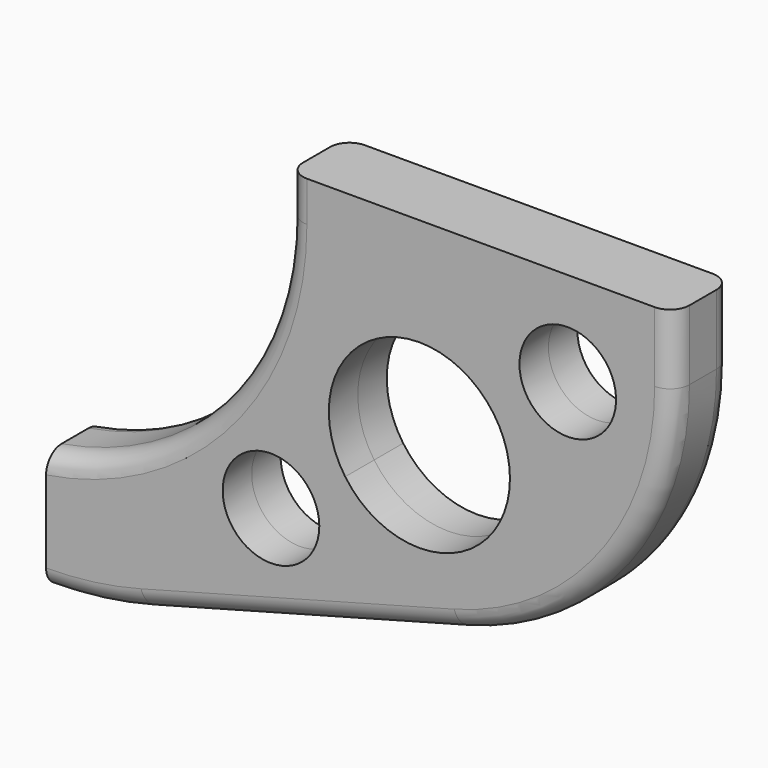
from build123d import *

# Parameters (mm, degrees)
F1_DEPTH = 9.525
F2_R     = 5.08


# Not quite as in the source:
# - a feature names something its author has since deleted; it is built from what else it names


with BuildPart() as f1:
    # F0 (on Front) → F1 (new body, symmetric)
    with BuildSketch(Plane.XZ):
        with BuildLine():
            Line((0, 15.875), (0, 0))
            ThreePointArc((0, 0), (13.2614611296, 0.8692020844), (26.2960149824, 3.461936049))
            Line((26.2960149824, 3.461936049), (108.6220112368, 25.5211202615))
            ThreePointArc((108.6220112368, 25.5211202615), (149.3535245302, 52.7370473342), (165.1, 99.1246682247))
            Line((165.1, 99.1246682247), (165.1, 117.475))
            Line((165.1, 117.475), (63.5, 117.475))
            Line((63.5, 117.475), (63.5, 106.8842132454))
            ThreePointArc((63.5, 106.8842132454), (45.4987113259, 57.6973247485), (0, 31.75))
            Line((0, 31.75), (0, 15.875))
        make_face()
        with BuildLine():
            ThreePointArc((71.8357677815, 38.1), (47.023562507, 34.2810363463), (69.5389987439, 45.3844207417))
            ThreePointArc((69.5389987439, 45.3844207417), (71.247973056, 41.9189636537), (71.8357677815, 38.1))
        make_face(mode=Mode.SUBTRACT)
        with BuildLine():
            ThreePointArc((117.6539419454, 79.0748666718), (120.8582687804, 72.5771346319), (121.9603838907, 65.4165777812))
            ThreePointArc((121.9603838907, 65.4165777812), (105.3084407414, 42.7061928915), (78.6418258361, 51.7582888906))
            ThreePointArc((78.6418258361, 51.7582888906), (84.4895950001, 84.9226358359), (117.6539419454, 79.0748666718))
        make_face(mode=Mode.SUBTRACT)
        with BuildLine():
            ThreePointArc((149.86, 92.7331555624), (140.9789636537, 80.6209502879), (126.7567690375, 85.4487348208))
            ThreePointArc((126.7567690375, 85.4487348208), (133.3410363463, 104.8453608369), (149.86, 92.7331555624))
        make_face(mode=Mode.SUBTRACT)
    extrude(amount=F1_DEPTH, both=True)

    # F2
    f2_edges = [f1.edges().sort_by_distance(p)[0] for p in [
        (45.498711, -9.525, 57.697325),
        (63.5, -9.525, 112.179607),
        (63.5, 9.525, 112.179607),
        (165.1, -9.525, 108.299834),
        (149.353525, -9.525, 52.737047),
        (13.261461, 9.525, 0.869202),
    ]]
    fillet(f2_edges, radius=F2_R)


solid = f1.part
